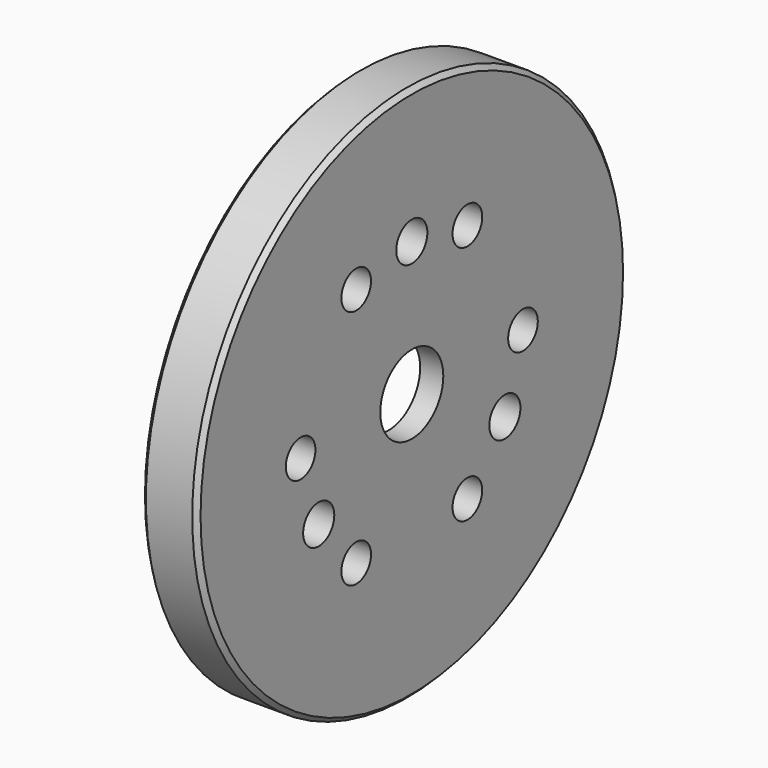
from build123d import *

# Parameters (mm, degrees)
F0_R     = 29
F0_R_2   = 2
F0_R_3   = 2.1
F0_R_4   = 4.25
F1_DEPTH = 6
F2_R     = 11
F3_DEPTH = 3.5
F4_SIZE  = 0.5


# Not quite as in the source:
# - a feature names something its author has since deleted; it is built from what else it names


with BuildPart() as f1:
    # F0 (on Right) → F1 (new body)
    with BuildSketch(Plane.YZ):
        Circle(F0_R)
        with Locations((-7.5, -12.9903810568)):
            Circle(F0_R_2, mode=Mode.SUBTRACT)
        with Locations((-12.5573683549, -7.25)):
            Circle(F0_R_3, mode=Mode.SUBTRACT)
        with Locations((7.5, -12.9903810568)):
            Circle(F0_R_2, mode=Mode.SUBTRACT)
        with Locations((12.5573683549, -7.25)):
            Circle(F0_R_3, mode=Mode.SUBTRACT)
        with Locations((-15, 0)):
            Circle(F0_R_2, mode=Mode.SUBTRACT)
        with Locations((-7.5, 12.9903810568)):
            Circle(F0_R_2, mode=Mode.SUBTRACT)
        Circle(F0_R_4, mode=Mode.SUBTRACT)
        with Locations((7.5, 12.9903810568)):
            Circle(F0_R_2, mode=Mode.SUBTRACT)
        with Locations((15, 0)):
            Circle(F0_R_2, mode=Mode.SUBTRACT)
        with Locations((0, 14.5)):
            Circle(F0_R_3, mode=Mode.SUBTRACT)
    extrude(amount=F1_DEPTH)

    # F2 (on Right) → F3 (cut)
    with BuildSketch(Plane.YZ):
        Circle(F2_R)
    extrude(amount=F3_DEPTH, mode=Mode.SUBTRACT)

    # F4
    f4_edges = [f1.edges().sort_by_distance(p)[0] for p in [
        (0, -11, 0),
        (0, -29, 0),
        (6, -29, 0),
    ]]
    chamfer(f4_edges, length=F4_SIZE)


solid = f1.part
